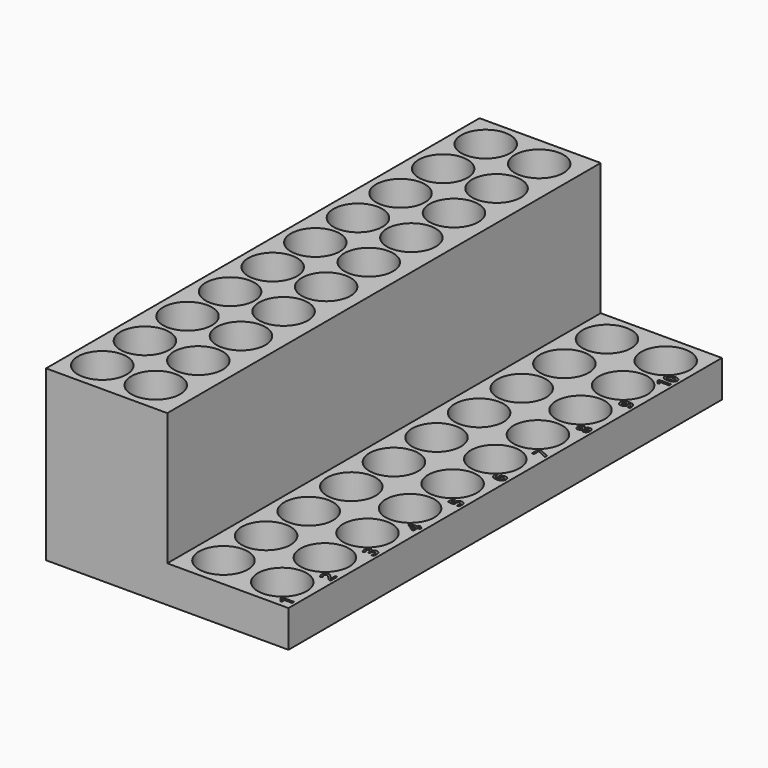
from build123d import *

# Parameters (mm, degrees)
F0_W         = 66
F0_H         = 20
F1_DEPTH     = 295
F2_R         = 13.3
F3_DEPTH     = 18
F5_DEPTH     = 295
F6_R         = 13.3
F7_DEPTH     = 18
F2_TEXT_SIZE = 9.1401168902
F8_DEPTH     = 18


# Not quite as in the source:
# - Text() gives the source's letters only with a copy of the font that has no kerning and outlines rounded to 1/6400 em; it was checked with that copy


with BuildPart() as f1:
    # F0 (on Front) → F1 (new body)
    with BuildSketch(Plane.XZ):
        with Locations((4.2099114507, -30.2171953642)):
            Rectangle(F0_W, F0_H)
    extrude(amount=-F1_DEPTH)

    # F2 (on face) → F3 (cut)
    with BuildSketch(Plane.XY.offset(-20.2171953642)):
        with Locations((-11.7900885493, 17)):
            Circle(F2_R)
        with Locations((-11.7900885493, 46)):
            Circle(F2_R)
        with Locations((-11.7900885493, 75)):
            Circle(F2_R)
        with Locations((-11.7900885493, 104)):
            Circle(F2_R)
        with Locations((-11.7900885493, 133)):
            Circle(F2_R)
        with Locations((-11.7900885493, 162)):
            Circle(F2_R)
        with Locations((-11.7900885493, 191)):
            Circle(F2_R)
        with Locations((-11.7900885493, 220)):
            Circle(F2_R)
        with Locations((-11.7900885493, 249)):
            Circle(F2_R)
        with Locations((-11.7900885493, 278)):
            Circle(F2_R)
        with Locations((20.2099114507, 278)):
            Circle(F2_R)
        with Locations((20.2099114507, 249)):
            Circle(F2_R)
        with Locations((20.2099114507, 220)):
            Circle(F2_R)
        with Locations((20.2099114507, 191)):
            Circle(F2_R)
        with Locations((20.2099114507, 162)):
            Circle(F2_R)
        with Locations((20.2099114507, 133)):
            Circle(F2_R)
        with Locations((20.2099114507, 104)):
            Circle(F2_R)
        with Locations((20.2099114507, 75)):
            Circle(F2_R)
        with Locations((20.2099114507, 46)):
            Circle(F2_R)
        with Locations((20.2099114507, 17)):
            Circle(F2_R)
    extrude(amount=-F3_DEPTH, mode=Mode.SUBTRACT)

    # F4 (on face) → F5 (join)
    with BuildSketch(Plane.XZ):
        Polygon((-28.7900885493, -40.2171953642), (-28.7900885493, -20.2171953642), (-28.7900885493, 51.7828046358), (-94.7900885493, 51.7828046358), (-94.7900885493, -40.2171953642), align=None)
    extrude(amount=-F5_DEPTH)

    # F6 (on face) → F7 (cut)
    with BuildSketch(Plane.XY.offset(51.7828046358)):
        with Locations((-77.7900885493, 17)):
            Circle(F6_R)
        with Locations((-48.689588502, 17)):
            Circle(F6_R)
        with Locations((-77.7900885493, 46)):
            Circle(F6_R)
        with Locations((-48.689588502, 46)):
            Circle(F6_R)
        with Locations((-48.689588502, 75)):
            Circle(F6_R)
        with Locations((-77.7900885493, 75)):
            Circle(F6_R)
        with Locations((-48.689588502, 104)):
            Circle(F6_R)
        with Locations((-77.7900885493, 104)):
            Circle(F6_R)
        with Locations((-48.689588502, 133)):
            Circle(F6_R)
        with Locations((-77.7900885493, 133)):
            Circle(F6_R)
        with Locations((-48.689588502, 162)):
            Circle(F6_R)
        with Locations((-77.7900885493, 162)):
            Circle(F6_R)
        with Locations((-48.689588502, 191)):
            Circle(F6_R)
        with Locations((-77.7900885493, 191)):
            Circle(F6_R)
        with Locations((-48.689588502, 220)):
            Circle(F6_R)
        with Locations((-77.7900885493, 220)):
            Circle(F6_R)
        with Locations((-48.689588502, 249)):
            Circle(F6_R)
        with Locations((-77.7900885493, 249)):
            Circle(F6_R)
        with Locations((-48.689588502, 278)):
            Circle(F6_R)
        with Locations((-77.7900885493, 278)):
            Circle(F6_R)
    extrude(amount=-F7_DEPTH, mode=Mode.SUBTRACT)

    # F2 (on face) → F8 (cut)
    with BuildSketch(Plane.XY.offset(-20.2171953642)):
        with Locations((-11.7900885493, 17)):
            Circle(F2_R)
        with Locations((20.2099114507, 17)):
            Circle(F2_R)
        with Locations((-11.7900885493, 46)):
            Circle(F2_R)
        with Locations((20.2099114507, 46)):
            Circle(F2_R)
        with Locations((-11.7900885493, 75)):
            Circle(F2_R)
        with Locations((20.2099114507, 75)):
            Circle(F2_R)
        with Locations((-11.7900885493, 104)):
            Circle(F2_R)
        with Locations((20.2099114507, 104)):
            Circle(F2_R)
        with Locations((-11.7900885493, 133)):
            Circle(F2_R)
        with Locations((20.2099114507, 133)):
            Circle(F2_R)
        with Locations((-11.7900885493, 162)):
            Circle(F2_R)
        with Locations((20.2099114507, 162)):
            Circle(F2_R)
        with Locations((-11.7900885493, 191)):
            Circle(F2_R)
        with Locations((20.2099114507, 191)):
            Circle(F2_R)
        with Locations((-11.7900885493, 220)):
            Circle(F2_R)
        with Locations((20.2099114507, 220)):
            Circle(F2_R)
        with Locations((-11.7900885493, 249)):
            Circle(F2_R)
        with Locations((20.2099114507, 249)):
            Circle(F2_R)
        with Locations((-11.7900885493, 278)):
            Circle(F2_R)
        with Locations((20.2099114507, 278)):
            Circle(F2_R)
        with Locations(Location((35.4704628116, 2.237487759), (0, 0, 90))):
            Text('1', F2_TEXT_SIZE, font='Open Sans', font_style=FontStyle.BOLD, text_align=(TextAlign.LEFT, TextAlign.BOTTOM))
        with Locations(Location((35.4704628116, 88.8006465393), (0, 0, 90))):
            Text('4', F2_TEXT_SIZE, font='Open Sans', font_style=FontStyle.BOLD, text_align=(TextAlign.LEFT, TextAlign.BOTTOM))
        with Locations(Location((35.4704628116, 59.7104115295), (0, 0, 90))):
            Text('3', F2_TEXT_SIZE, font='Open Sans', font_style=FontStyle.BOLD, text_align=(TextAlign.LEFT, TextAlign.BOTTOM))
        with Locations(Location((35.4704628116, 30.49584775), (0, 0, 90))):
            Text('2', F2_TEXT_SIZE, font='Open Sans', font_style=FontStyle.BOLD, text_align=(TextAlign.LEFT, TextAlign.BOTTOM))
        with Locations(Location((35.4704628116, 117.908172484), (0, 0, 90))):
            Text('5', F2_TEXT_SIZE, font='Open Sans', font_style=FontStyle.BOLD, text_align=(TextAlign.LEFT, TextAlign.BOTTOM))
        with Locations(Location((35.4704628116, 147.3951080698), (0, 0, 90))):
            Text('6', F2_TEXT_SIZE, font='Open Sans', font_style=FontStyle.BOLD, text_align=(TextAlign.LEFT, TextAlign.BOTTOM))
        with Locations(Location((35.4704628116, 175.7330784458), (0, 0, 90))):
            Text('7', F2_TEXT_SIZE, font='Open Sans', font_style=FontStyle.BOLD, text_align=(TextAlign.LEFT, TextAlign.BOTTOM))
        with Locations(Location((35.4704628116, 204.7235557693), (0, 0, 90))):
            Text('8', F2_TEXT_SIZE, font='Open Sans', font_style=FontStyle.BOLD, text_align=(TextAlign.LEFT, TextAlign.BOTTOM))
        with Locations(Location((35.4704628116, 233.7227502721), (0, 0, 90))):
            Text('9', F2_TEXT_SIZE, font='Open Sans', font_style=FontStyle.BOLD, text_align=(TextAlign.LEFT, TextAlign.BOTTOM))
        with Locations(Location((35.4704628116, 258.7951609748), (0, 0, 90))):
            Text('10', F2_TEXT_SIZE, font='Open Sans', font_style=FontStyle.BOLD, text_align=(TextAlign.LEFT, TextAlign.BOTTOM))
    extrude(amount=-F8_DEPTH, mode=Mode.SUBTRACT)


solid = f1.part
